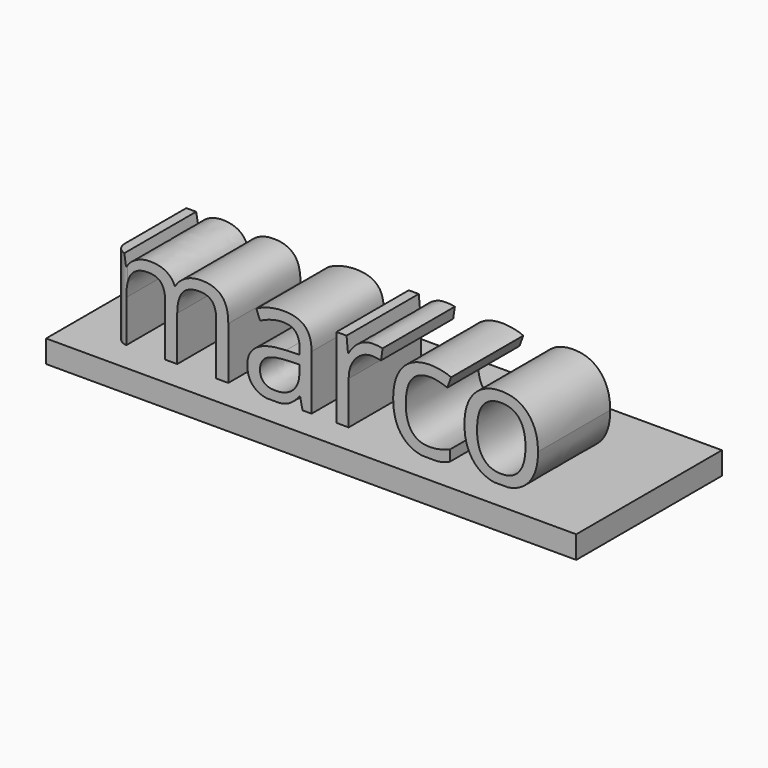
from build123d import *

# Parameters (mm, degrees)
F0_W         = 117.4760833383
F0_H         = 40.3480958194
F1_DEPTH     = 5
F2_TEXT_SIZE = 33.1659542604
F3_DEPTH     = 20
F4_R         = 3


# Not quite as in the source:
# - Text() gives the source's letters only with a copy of the font that has no kerning and outlines rounded to 1/6400 em; it was checked with that copy


with BuildPart() as f1:
    # F0 (on Top) → F1 (new body)
    with BuildSketch(Plane.XY):
        with Locations((1.7840974033, -6.1757294461)):
            Rectangle(F0_W, F0_H)
    extrude(amount=F1_DEPTH)

    # F2 (on Front) → F3 (join)
    with BuildSketch(Plane.XZ):
        with Locations((-49.8175472021, 5.2150599658)):
            Text('marco', F2_TEXT_SIZE, font='Open Sans', text_align=(TextAlign.LEFT, TextAlign.BOTTOM))
    extrude(amount=F3_DEPTH)

    # F4
    f4_edges = [f1.edges().sort_by_distance(p)[0] for p in [
        (-46.967348, -20, 14.089544),
    ]]
    fillet(f4_edges, radius=F4_R)


solid = f1.part
